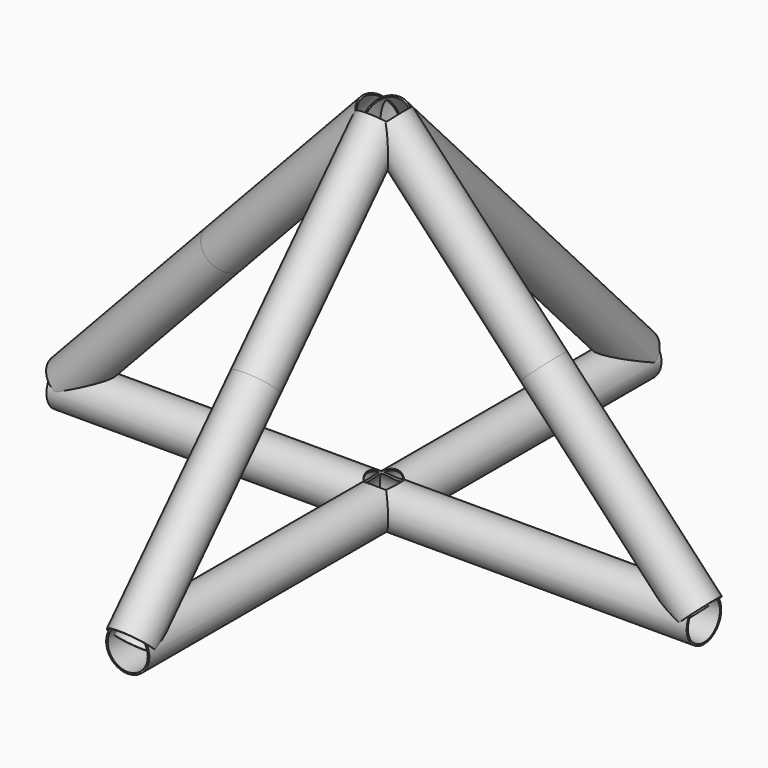
from build123d import *

# Parameters (mm, degrees)
F2_R           = 13.5
F2_R_2         = 12.5
F3_DEPTH       = 200
F3_DEPTH_BACK  = 200
F4_R           = 13.5
F4_R_2         = 12.5
F5_DEPTH       = 200
F5_DEPTH_BACK  = 200
F12_R          = 13.5
F12_R_2        = 12.5
F13_DEPTH      = 141.4
F13_DEPTH_BACK = 141.4
F14_R          = 13.5
F14_R_2        = 12.5
F15_DEPTH      = 141.4
F15_DEPTH_BACK = 141.4
F16_R          = 13.5
F16_R_2        = 12.5
F17_DEPTH      = 141.4
F17_DEPTH_BACK = 141.4
F18_R          = 13.5
F18_R_2        = 12.5
F19_DEPTH      = 141.4
F19_DEPTH_BACK = 141.4
F20_R          = 10
F21_DEPTH      = 50


# Not quite as in the source:
# - the program builds the solid bodies; features that only make, move or delete a surface that nothing else refers to are left out


with BuildPart() as f3:
    # F2 (on Front) → F3 (new body, two sides)
    with BuildSketch(Plane.XZ) as f3_sk:
        Circle(F2_R)
        Circle(F2_R_2, mode=Mode.SUBTRACT)
    extrude(amount=-F3_DEPTH)
    extrude(f3_sk.sketch, amount=F3_DEPTH_BACK)

    # F4 (on Right) → F5 (join, two sides)
    with BuildSketch(Plane.YZ) as f5_sk:
        Circle(F4_R)
        Circle(F4_R_2, mode=Mode.SUBTRACT)
    extrude(amount=F5_DEPTH)
    extrude(f5_sk.sketch, amount=-F5_DEPTH_BACK)

    # F12 (on line) → F13 (join, two sides)
    with BuildSketch(Plane(origin=(0, -6.1925362702, 6.5877968823), x_dir=(1, 0, 0), z_dir=(0, -0.6849104316, 0.7286272714))) as f13_sk:
        with Locations((0, 144.5252299309)):
            Circle(F12_R)
        with Locations((0, 144.5252299309)):
            Circle(F12_R_2, mode=Mode.SUBTRACT)
    extrude(amount=F13_DEPTH)
    extrude(f13_sk.sketch, amount=-F13_DEPTH_BACK)

    # F14 (on line) → F15 (join, two sides)
    with BuildSketch(Plane(origin=(6.6960868612, 0, 7.1613197136), x_dir=(0.7304348481, 0, -0.682982381), z_dir=(-0.682982381, 0, -0.7304348481))) as f15_sk:
        with Locations((-145.8499282598, 0)):
            Circle(F14_R)
        with Locations((-145.8499282598, 0)):
            Circle(F14_R_2, mode=Mode.SUBTRACT)
    extrude(amount=F15_DEPTH)
    extrude(f15_sk.sketch, amount=-F15_DEPTH_BACK)

    # F16 (on line) → F17 (join, two sides)
    with BuildSketch(Plane(origin=(-6.6447982018, 0, 7.1025389191), x_dir=(0.7302464024, 0, 0.6831838638), z_dir=(-0.6831838638, 0, 0.7302464024))) as f17_sk:
        with Locations((146.0631936789, 0)):
            Circle(F16_R)
        with Locations((146.0631936789, 0)):
            Circle(F16_R_2, mode=Mode.SUBTRACT)
    extrude(amount=F17_DEPTH)
    extrude(f17_sk.sketch, amount=-F17_DEPTH_BACK)

    # F18 (on line) → F19 (join, two sides)
    with BuildSketch(Plane(origin=(0, 6.3086895458, 6.719705981), x_dir=(1, 0, 0), z_dir=(0, -0.6844586379, -0.7290516944))) as f19_sk:
        with Locations((0, 145.9031552076)):
            Circle(F18_R)
        with Locations((0, 145.9031552076)):
            Circle(F18_R_2, mode=Mode.SUBTRACT)
    extrude(amount=F19_DEPTH)
    extrude(f19_sk.sketch, amount=-F19_DEPTH_BACK)

    # F20 (on Top) → F21 (cut)
    with BuildSketch(Plane.XY):
        Circle(F20_R)
    extrude(amount=F21_DEPTH, mode=Mode.SUBTRACT)


solid = f3.part
